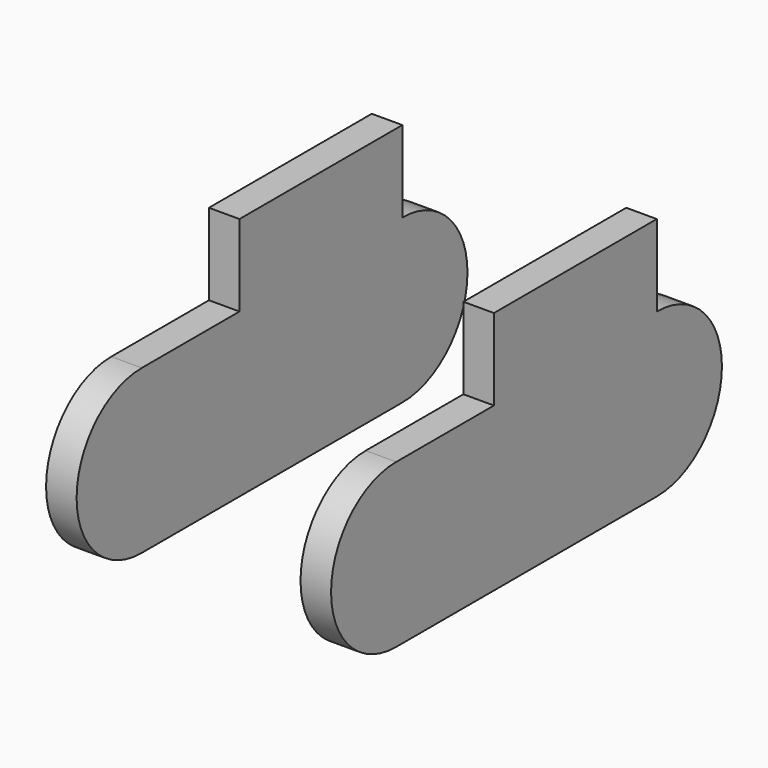
from build123d import *

# Parameters (mm, degrees)
F0_R     = 3
F0_W     = 20
F0_H     = 8
F1_DEPTH = 3


# Not quite as in the source:
# - a feature names something its author has since deleted; it is built from what else it names


with BuildPart() as f1:
    # F0 (on Right) → F1 (new body)
    with BuildSketch(Plane.YZ):
        with BuildLine():
            ThreePointArc((-18.3839101195, 17.088659659), (-26.3839101195, 9.088659659), (-18.3839101195, 1.088659659))
            Line((-18.3839101195, 1.088659659), (13.6160898805, 1.088659659))
            ThreePointArc((13.6160898805, 1.088659659), (21.6160898805, 9.088659659), (13.6160898805, 17.088659659))
            Line((13.6160898805, 17.088659659), (-6.3839101195, 17.088659659))
            Line((-6.3839101195, 17.088659659), (-18.3839101195, 17.088659659))
        make_face()
        with Locations((-18.3839101195, 9.088659659)):
            Circle(F0_R, mode=Mode.SUBTRACT)
        with Locations((13.6160898805, 9.088659659)):
            Circle(F0_R, mode=Mode.SUBTRACT)
        with Locations((3.6160898805, 21.088659659)):
            Rectangle(F0_W, F0_H)
        with Locations((-18.3839101195, 9.088659659)):
            Circle(F0_R)
        with Locations((13.6160898805, 9.088659659)):
            Circle(F0_R)
    extrude(amount=F1_DEPTH)


with BuildPart() as f4_1:
    # F4: instance of F1
    add(f1.part.mirror(Plane(origin=(-11, 3.6160898805, 23.588659659), x_dir=(0, -1, 0), z_dir=(1, 0, 0))))


solid = Compound([f1.part, f4_1.part])
